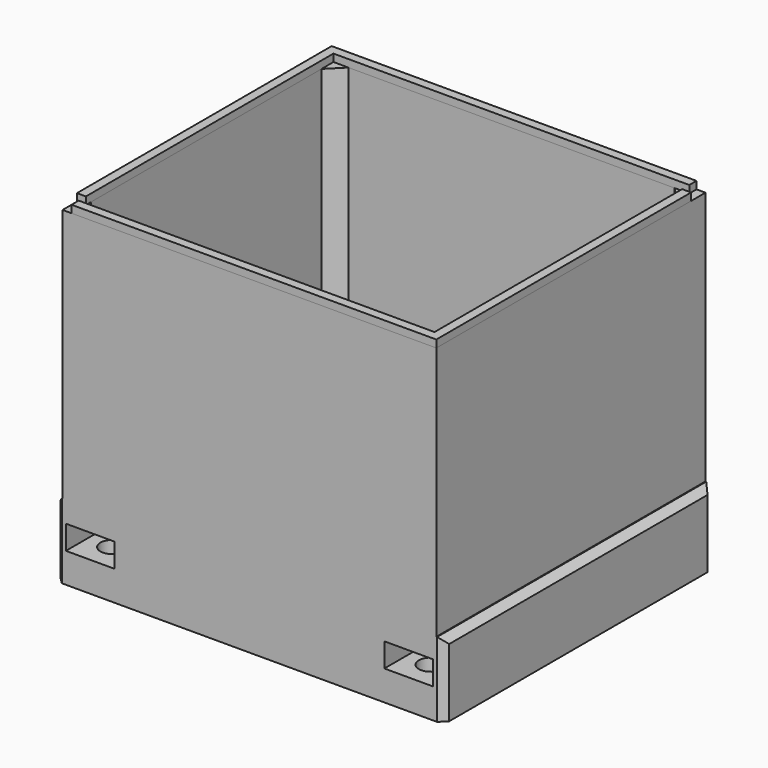
from build123d import *

# Parameters (mm, degrees)
F0_W      = 47.6
F0_H      = 1.2
F0_W_2    = 1.2
F0_H_2    = 42.6
F1_DEPTH  = 44
F2_R      = 1.6
F2_W      = 1.4791749234
F2_H      = 26.2
F2_W_2    = 2.291076839
F3_DEPTH  = 10
F4_W      = 6.5
F4_H      = 3.2
F5_DEPTH  = 7.1
F6_START  = -37.9
F6_DEPTH  = 7.1
F7_SIZE   = 0.9
F8_W      = 47.6
F8_H      = 1.2
F8_W_2    = 1.2
F8_H_2    = 41.4
F9_DEPTH  = 1
F10_W     = 33.2
F10_H     = 5
F11_DEPTH = 8
F12_SIZE  = 1.99999
F13_SIZE  = 2
F14_SIZE  = 1.2


# Not quite as in the source:
# - a fillet or chamfer is up to 0.001 mm smaller than in the source, because OpenCascade refuses the exact size


with BuildPart() as f1:
    # F0 (on Top) → F1 (new body)
    with BuildSketch(Plane.XY):
        with Locations((25, 44.4)):
            Rectangle(F0_W, F0_H)
        with Locations((49.4, 44.4)):
            Rectangle(F0_W_2, F0_H)
        with Locations((49.4, 22.5)):
            Rectangle(F0_W_2, F0_H_2)
        with Locations((49.4, 0.6)):
            Rectangle(F0_W_2, F0_H)
        with Locations((25, 0.6)):
            Rectangle(F0_W, F0_H)
        with Locations((0.6, 0.6)):
            Rectangle(F0_W_2, F0_H)
        with Locations((0.6, 22.5)):
            Rectangle(F0_W_2, F0_H_2)
        with Locations((0.6, 44.4)):
            Rectangle(F0_W_2, F0_H)
    extrude(amount=F1_DEPTH)

    # F2 (on face) → F3 (join)
    with BuildSketch(Plane.XY):
        Polygon((-1, 9.4), (-1, 0), (8.4, 0), (8.4, 9.4), (0.4791749234, 9.4), align=None)
        with Locations((3.7, 3.7)):
            Circle(F2_R, mode=Mode.SUBTRACT)
        with Locations((-0.2604125383, 22.5)):
            Rectangle(F2_W, F2_H)
        Polygon((-1, 45), (-1, 35.6), (0.4791749234, 35.6), (8.4, 35.6), (8.4, 45), align=None)
        with Locations((3.7, 41.3)):
            Circle(F2_R, mode=Mode.SUBTRACT)
        Polygon((41.6, 9.4), (41.6, 0), (51, 0), (51, 9.4), (48.708923161, 9.4), align=None)
        with Locations((46.3, 3.7)):
            Circle(F2_R, mode=Mode.SUBTRACT)
        with Locations((49.8544615805, 22.5)):
            Rectangle(F2_W_2, F2_H)
        Polygon((41.6, 35.6), (48.708923161, 35.6), (51, 35.6), (51, 45), (41.6, 45), align=None)
        with Locations((46.3, 41.3)):
            Circle(F2_R, mode=Mode.SUBTRACT)
    extrude(amount=F3_DEPTH)

    # F4 (on face) → F5 (cut)
    with BuildSketch(Plane.XZ):
        with Locations((3.7, 5.6)):
            Rectangle(F4_W, F4_H)
        with Locations((46.3, 5.6)):
            Rectangle(F4_W, F4_H)
    extrude(amount=-F5_DEPTH, mode=Mode.SUBTRACT)

    # F4 (on face) → F6 (cut)
    with BuildSketch(Plane.XZ.offset(F6_START)):
        with Locations((3.7, 5.6)):
            Rectangle(F4_W, F4_H)
        with Locations((46.3, 5.6)):
            Rectangle(F4_W, F4_H)
    extrude(amount=-F6_DEPTH, mode=Mode.SUBTRACT)

    # F7
    f7_edges = [f1.edges().sort_by_distance(p)[0] for p in [
        (-1, 45, 5),
        (-1, 22.5, 10),
        (51, 22.5, 10),
        (-1, 0, 5),
        (51, 0, 5),
        (51, 45, 5),
    ]]
    chamfer(f7_edges, length=F7_SIZE)

    # F10 (on face) → F11 (join)
    with BuildSketch(Plane.XY):
        with Locations((25, 41.3)):
            Rectangle(F10_W, F10_H)
        with Locations((25, 3.7)):
            Rectangle(F10_W, F10_H)
    extrude(amount=F11_DEPTH)

    # F12 (size 2 in the source; OpenCascade refuses exactly that, so slightly less here)
    f12_edges = [f1.edges().sort_by_distance(p)[0] for p in [
        (8.4, 41.3, 8),
        (41.6, 41.3, 8),
        (41.6, 38.8, 4),
        (8.4, 38.8, 4),
        (41.6, 6.2, 4),
        (41.6, 3.7, 8),
        (8.4, 3.7, 8),
        (8.4, 6.2, 4),
        (1.2, 35.6, 5),
        (48.708923, 35.6, 5),
        (48.708923, 9.4, 5),
        (1.2, 9.4, 5),
    ]]
    chamfer(f12_edges, length=F12_SIZE)

    # F13
    f13_edges = [f1.edges().sort_by_distance(p)[0] for p in [
        (48.8, 43.8, 27),
        (1.2, 43.8, 27),
        (1.2, 1.2, 27),
        (48.8, 1.2, 27),
    ]]
    chamfer(f13_edges, length=F13_SIZE)

    # F14
    f14_edges = [f1.edges().sort_by_distance(p)[0] for p in [
        (8.4, 35.6, 5),
        (41.6, 35.6, 5),
        (41.6, 9.4, 5),
        (8.4, 9.4, 5),
    ]]
    chamfer(f14_edges, length=F14_SIZE)


with BuildPart() as f9:
    # F8 (on face) → F9 (new body)
    with BuildSketch(Plane.XY.offset(44)):
        with Locations((25, 44.4)):
            Rectangle(F8_W, F8_H)
        with Locations((0.6, 23.1)):
            Rectangle(F8_W_2, F8_H_2)
        with Locations((0.6, 44.4)):
            Rectangle(F8_W_2, F8_H)
    extrude(amount=F9_DEPTH)


with BuildPart() as f9b:
    # F8 (on face) → F9, piece 2 (new body)
    with BuildSketch(Plane.XY.offset(44)):
        with Locations((49.4, 21.9)):
            Rectangle(F8_W_2, F8_H_2)
        with Locations((25, 0.6)):
            Rectangle(F8_W, F8_H)
        with Locations((49.4, 0.6)):
            Rectangle(F8_W_2, F8_H)
    extrude(amount=F9_DEPTH)


solid = Compound([f1.part, f9.part, f9b.part])
